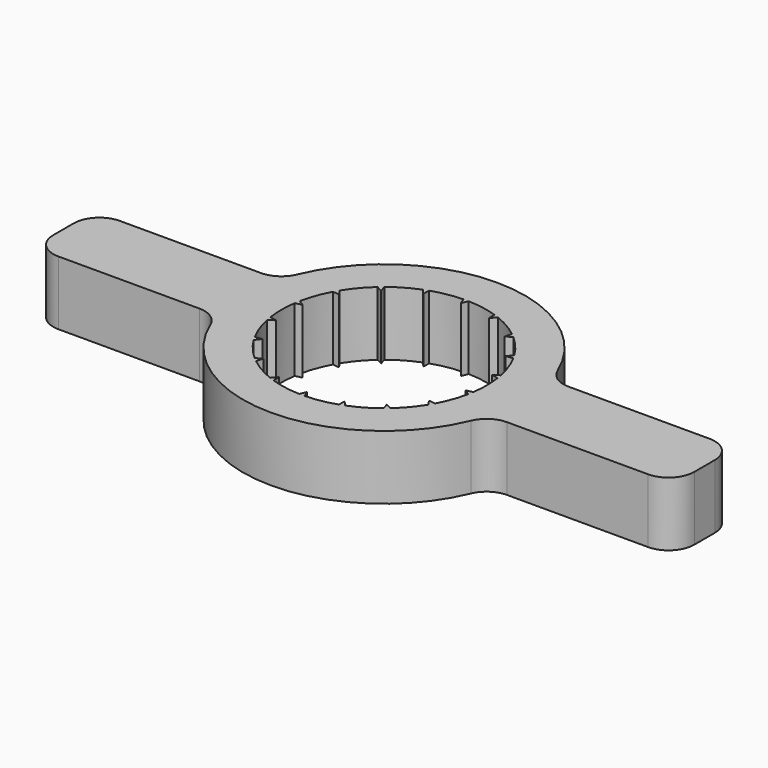
from build123d import *

# Parameters (mm, degrees)
F0_R            = 8
F1_DEPTH        = 5
F3_DEPTH        = 5
F3_COPIES_COUNT = 18
F4_R            = 2


# Not quite as in the source:
# - a pattern or mirror of a feature is missing from the dataset's text; its kind, count and spacing are read off the source's solid


with BuildPart() as f1:
    # F0 (on Top) → F1 (new body)
    with BuildSketch(Plane.XY):
        with BuildLine():
            Line((-25, -3), (-10.5830052443, -3))
            ThreePointArc((-10.5830052443, -3), (0, -11), (10.5830052443, -3))
            Line((10.5830052443, -3), (25, -3))
            Line((25, -3), (25, 3))
            Line((25, 3), (10.5830052443, 3))
            ThreePointArc((10.5830052443, 3), (0, 11), (-10.5830052443, 3))
            Line((-10.5830052443, 3), (-25, 3))
            Line((-25, 3), (-25, -3))
        make_face()
        Circle(F0_R, mode=Mode.SUBTRACT)
    extrude(amount=F1_DEPTH)

    # F2 (on Top) → F3 (join)
    with BuildSketch(Plane.XY):
        with BuildLine():
            Line((0, -7.5), (-0.2060079166, -7.9973471063))
            ThreePointArc((-0.2060079166, -7.9973471063), (0, -8), (0.2060079166, -7.9973471063))
            Line((0.2060079166, -7.9973471063), (0, -7.5))
        make_face()
    f3 = extrude(amount=F3_DEPTH)

    # F3_copies: F3 ×18 about axis
    f3_copies_axis = Axis((0, 0, 0), (0, 0, 1))
    for i in range(1, F3_COPIES_COUNT):
        add(f3.rotate(f3_copies_axis, i * 360 / F3_COPIES_COUNT))

    # F4
    f4_edges = [f1.edges().sort_by_distance(p)[0] for p in [
        (-25, 3, 2.5),
        (-25, -3, 2.5),
        (25, 3, 2.5),
        (-10.583005, 3, 2.5),
        (25, -3, 2.5),
        (10.583005, -3, 2.5),
        (-10.583005, -3, 2.5),
        (10.583005, 3, 2.5),
    ]]
    fillet(f4_edges, radius=F4_R)


solid = f1.part
